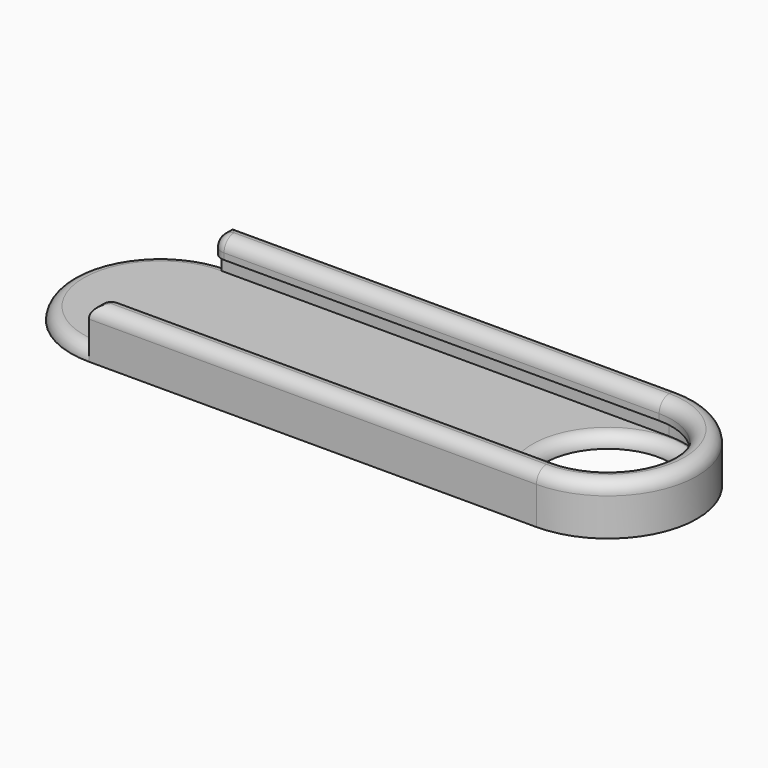
from build123d import *

# Parameters (mm, degrees)
F0_R         = 5
F1_DEPTH     = 1
F2_DEPTH     = 2.5
F4_DEPTH     = 1.5
F5_T1_DEPTH  = 35.75
F5_T3_DEPTH  = 1
F5_T5_DEPTH  = 34.75
F5_T7_DEPTH  = 1
F5_T9_DEPTH  = 0.5
F5_S13_W     = 1.02
F5_S13_H     = 1.02
F5_T14_DEPTH = 1.02
F5_S19_W     = 1.02
F5_S19_H     = 1.02
F5_T20_DEPTH = 1.02
F5_T24_ANGLE = 180
F5_T26_ANGLE = 180
F5_T30_ANGLE = 180
F5_T35_DEPTH = 3.5
F5_T39_DEPTH = 38.25
F5_T46_DEPTH = 38.25
F5_T50_DEPTH = 3.5


# Not quite as in the source:
# - a fillet or chamfer that OpenCascade refuses, or shapes differently, is made with other operations: its cross-section is extruded or revolved along the edge and cut away or added


with BuildPart() as f1:
    # F0 (on Top) → F1 (new body)
    with BuildSketch(Plane.XY):
        with BuildLine():
            Line((-12.4595724046, -6.125), (23.2904275954, -6.125))
            ThreePointArc((23.2904275954, -6.125), (29.4154275954, 0), (23.2904275954, 6.125))
            Line((23.2904275954, 6.125), (-12.4595724046, 6.125))
            ThreePointArc((-12.4595724046, 6.125), (-18.5845724046, 0), (-12.4595724046, -6.125))
        make_face()
        with Locations((23.2904275954, 0)):
            Circle(F0_R, mode=Mode.SUBTRACT)
        with BuildLine():
            Line((-12.4595724046, -7.125), (-12.4595724046, -6.125))
            ThreePointArc((-12.4595724046, -6.125), (-18.5845724046, 0), (-12.4595724046, 6.125))
            Line((-12.4595724046, 6.125), (-12.4595724046, 7.125))
            ThreePointArc((-12.4595724046, 7.125), (-19.5845724046, 0), (-12.4595724046, -7.125))
        make_face()
    extrude(amount=F1_DEPTH)

    # F0 (on Top) → F2 (join)
    with BuildSketch(Plane.XY):
        with BuildLine():
            ThreePointArc((23.2904275954, 6.125), (29.4154275954, 0), (23.2904275954, -6.125))
            Line((23.2904275954, -6.125), (-12.4595724046, -6.125))
            Line((-12.4595724046, -6.125), (-12.4595724046, -7.125))
            Line((-12.4595724046, -7.125), (23.2904275954, -7.125))
            ThreePointArc((23.2904275954, -7.125), (30.4154275954, 0), (23.2904275954, 7.125))
            Line((23.2904275954, 7.125), (-12.4595724046, 7.125))
            Line((-12.4595724046, 7.125), (-12.4595724046, 6.125))
            Line((-12.4595724046, 6.125), (23.2904275954, 6.125))
        make_face()
    extrude(amount=F2_DEPTH)

    # F3 (on face) → F4 (join)
    with BuildSketch(Plane.XY.offset(2.5)):
        with BuildLine():
            Line((-12.4595724046, -7.125), (23.2904275954, -7.125))
            ThreePointArc((23.2904275954, -7.125), (30.4154275954, 0), (23.2904275954, 7.125))
            Line((23.2904275954, 7.125), (-12.4595724046, 7.125))
            Line((-12.4595724046, 7.125), (-12.4595724046, 6.125))
            Line((-12.4595724046, 6.125), (23.2904275954, 6.125))
            ThreePointArc((23.2904275954, 6.125), (29.4154275954, 0), (23.2904275954, -6.125))
            Line((23.2904275954, -6.125), (-12.4595724046, -6.125))
            Line((-12.4595724046, -6.125), (-12.4595724046, -7.125))
        make_face()
        with BuildLine():
            Line((-12.4595724046, -5.125), (-12.4595724046, -6.125))
            Line((-12.4595724046, -6.125), (23.2904275954, -6.125))
            ThreePointArc((23.2904275954, -6.125), (29.4154275954, 0), (23.2904275954, 6.125))
            Line((23.2904275954, 6.125), (-12.4595724046, 6.125))
            Line((-12.4595724046, 6.125), (-12.4595724046, 5.125))
            Line((-12.4595724046, 5.125), (23.2904275954, 5.125))
            ThreePointArc((23.2904275954, 5.125), (28.4154275954, 0), (23.2904275954, -5.125))
            Line((23.2904275954, -5.125), (-12.4595724046, -5.125))
        make_face()
    extrude(amount=F4_DEPTH)

    # F5: fillet of radius 1 on 12 edges, made by hand

    # F5_s2 → F5_t1 (cut)
    with BuildSketch(Plane.YZ.offset(-12.4595724046)):
        with BuildLine():
            ThreePointArc((-6.125, 4), (-6.8321067812, 3.7071067812), (-7.125, 3))
            Line((-7.125, 3), (-7.145, 3))
            Line((-7.145, 3), (-7.145, 4.02))
            Line((-7.145, 4.02), (-6.125, 4.02))
            Line((-6.125, 4.02), (-6.125, 4))
        make_face()
        with BuildLine():
            ThreePointArc((6.125, 4), (6.8321067812, 3.7071067812), (7.125, 3))
            Line((7.125, 3), (7.145, 3))
            Line((7.145, 3), (7.145, 4.02))
            Line((7.145, 4.02), (6.125, 4.02))
            Line((6.125, 4.02), (6.125, 4))
        make_face()
    extrude(amount=F5_T1_DEPTH, mode=Mode.SUBTRACT)

    # F5_s4 → F5_t3 (cut)
    with BuildSketch(Plane.XZ.offset(-7.125)):
        with BuildLine():
            ThreePointArc((-11.4595724046, 4), (-12.1666791858, 3.7071067812), (-12.4595724046, 3))
            Line((-12.4595724046, 3), (-12.4795724046, 3))
            Line((-12.4795724046, 3), (-12.4795724046, 4.02))
            Line((-12.4795724046, 4.02), (-11.4595724046, 4.02))
            Line((-11.4595724046, 4.02), (-11.4595724046, 4))
        make_face()
    extrude(amount=F5_T3_DEPTH, mode=Mode.SUBTRACT)

    # F5_s6 → F5_t5 (cut)
    with BuildSketch(Plane.YZ.offset(-11.4595724046)):
        with BuildLine():
            ThreePointArc((6.125, 4), (5.4178932188, 3.7071067812), (5.125, 3))
            Line((5.125, 3), (5.105, 3))
            Line((5.105, 3), (5.105, 4.02))
            Line((5.105, 4.02), (6.125, 4.02))
            Line((6.125, 4.02), (6.125, 4))
        make_face()
        with BuildLine():
            ThreePointArc((-6.125, 4), (-5.4178932188, 3.7071067812), (-5.125, 3))
            Line((-5.125, 3), (-5.105, 3))
            Line((-5.105, 3), (-5.105, 4.02))
            Line((-5.105, 4.02), (-6.125, 4.02))
            Line((-6.125, 4.02), (-6.125, 4))
        make_face()
    extrude(amount=F5_T5_DEPTH, mode=Mode.SUBTRACT)

    # F5_s8 → F5_t7 (cut)
    with BuildSketch(Plane.XZ.offset(6.125)):
        with BuildLine():
            ThreePointArc((-12.4595724046, 3), (-12.1666791858, 3.7071067812), (-11.4595724046, 4))
            Line((-11.4595724046, 4), (-11.4595724046, 4.02))
            Line((-11.4595724046, 4.02), (-12.4795724046, 4.02))
            Line((-12.4795724046, 4.02), (-12.4795724046, 3))
            Line((-12.4795724046, 3), (-12.4595724046, 3))
        make_face()
    extrude(amount=F5_T7_DEPTH, mode=Mode.SUBTRACT)

    # F5_s10 → F5_t9 (cut)
    with BuildSketch(Plane.XY.offset(2.5)):
        with BuildLine():
            ThreePointArc((-12.4595724046, -6.125), (-12.1666791858, -5.4178932188), (-11.4595724046, -5.125))
            Line((-11.4595724046, -5.125), (-11.4595724046, -5.105))
            Line((-11.4595724046, -5.105), (-12.4795724046, -5.105))
            Line((-12.4795724046, -5.105), (-12.4795724046, -6.125))
            Line((-12.4795724046, -6.125), (-12.4595724046, -6.125))
        make_face()
        with BuildLine():
            ThreePointArc((-11.4595724046, 5.125), (-12.1666791858, 5.4178932188), (-12.4595724046, 6.125))
            Line((-12.4595724046, 6.125), (-12.4795724046, 6.125))
            Line((-12.4795724046, 6.125), (-12.4795724046, 5.105))
            Line((-12.4795724046, 5.105), (-11.4595724046, 5.105))
            Line((-11.4595724046, 5.105), (-11.4595724046, 5.125))
        make_face()
    extrude(amount=F5_T9_DEPTH, mode=Mode.SUBTRACT)


with BuildPart() as f5_tool12:
    # F5_s13 → F5_t14 (new body)
    with BuildSketch(Plane.YZ.offset(-11.4595724046)):
        with Locations((5.615, 3.51)):
            Rectangle(F5_S13_W, F5_S13_H)
    extrude(amount=-F5_T14_DEPTH)

    # F5_s15 → F5_t16 (revolve, cut)
    with BuildSketch(Plane(origin=(-11.4595724046, 6.125, 3), x_dir=(0, 0.7071067812, -0.7071067812), z_dir=(0, 0.7071067812, 0.7071067812))):
        with BuildLine():
            ThreePointArc((0, -1), (1, 0), (0, 1))
            Line((0, 1), (0, -1))
        make_face()
    revolve(axis=Axis((-11.4595724046, 6.125, 3), (-1, 0, 0)), mode=Mode.SUBTRACT)


with BuildPart() as f1_1:
    add(f1.part)

    # F5_t11: cut F5_tool12
    add(f5_tool12.part, mode=Mode.SUBTRACT)


with BuildPart() as f5_tool18:
    # F5_s19 → F5_t20 (new body)
    with BuildSketch(Plane.XZ.offset(6.125)):
        with Locations((-11.9695724046, 3.51)):
            Rectangle(F5_S19_W, F5_S19_H)
    extrude(amount=-F5_T20_DEPTH)

    # F5_s21 → F5_t22 (revolve, cut)
    with BuildSketch(Plane(origin=(-11.4595724046, -6.125, 3), x_dir=(0.7071067812, 0, -0.7071067812), z_dir=(0.7071067812, 0, 0.7071067812))):
        with BuildLine():
            ThreePointArc((0, -1), (1, 0), (0, 1))
            Line((0, 1), (0, -1))
        make_face()
    revolve(axis=Axis((-11.4595724046, -6.125, 3), (0, 1, 0)), mode=Mode.SUBTRACT)


with BuildPart() as f1_2:
    add(f1_1.part)

    # F5_t17: cut F5_tool18
    add(f5_tool18.part, mode=Mode.SUBTRACT)

    # F5_s23 → F5_t24 (revolve, cut)
    with BuildSketch(Plane.YZ.offset(23.2904275954)):
        with BuildLine():
            ThreePointArc((-6.125, 4), (-6.8321067812, 3.7071067812), (-7.125, 3))
            Line((-7.125, 3), (-7.145, 3))
            Line((-7.145, 3), (-7.145, 4.02))
            Line((-7.145, 4.02), (-6.125, 4.02))
            Line((-6.125, 4.02), (-6.125, 4))
        make_face()
    revolve(axis=Axis((23.2904275954, 0, 4), (0, 0, 1)), revolution_arc=F5_T24_ANGLE, mode=Mode.SUBTRACT)

    # F5_s25 → F5_t26 (revolve, cut)
    with BuildSketch(Plane.YZ.offset(23.2904275954)):
        with BuildLine():
            ThreePointArc((6.125, 4), (5.4178932188, 3.7071067812), (5.125, 3))
            Line((5.125, 3), (5.105, 3))
            Line((5.105, 3), (5.105, 4.02))
            Line((5.105, 4.02), (6.125, 4.02))
            Line((6.125, 4.02), (6.125, 4))
        make_face()
    revolve(axis=Axis((23.2904275954, 0, 4), (0, 0, -1)), revolution_arc=F5_T26_ANGLE, mode=Mode.SUBTRACT)

    # F5_s27 → F5_t28 (revolve, cut)
    with BuildSketch(Plane.XZ):
        with BuildLine():
            ThreePointArc((29.2904275954, 1), (28.5833208142, 0.7071067812), (28.2904275954, 0))
            Line((28.2904275954, 0), (28.2704275954, 0))
            Line((28.2704275954, 0), (28.2704275954, 1.02))
            Line((28.2704275954, 1.02), (29.2904275954, 1.02))
            Line((29.2904275954, 1.02), (29.2904275954, 1))
        make_face()
    revolve(axis=Axis((23.2904275954, 0, 1), (0, 0, 1)), mode=Mode.SUBTRACT)

    # F5_s29 → F5_t30 (revolve, cut)
    with BuildSketch(Plane.YZ.offset(-12.4595724046)):
        with BuildLine():
            ThreePointArc((7.125, 0), (6.8321067812, 0.7071067812), (6.125, 1))
            Line((6.125, 1), (6.125, 1.02))
            Line((6.125, 1.02), (7.145, 1.02))
            Line((7.145, 1.02), (7.145, 0))
            Line((7.145, 0), (7.125, 0))
        make_face()
    revolve(axis=Axis((-12.4595724046, 0, 1), (0, 0, 1)), revolution_arc=F5_T30_ANGLE, mode=Mode.SUBTRACT)


with BuildPart() as f5_tool33:
    # F5_s34 → F5_t35 (new body)
    with BuildSketch(Plane.XZ.offset(6.125)):
        with BuildLine():
            ThreePointArc((-12.4595724046, 3), (-12.1666791858, 3.7071067812), (-11.4595724046, 4))
            Line((-11.4595724046, 4), (-11.4595724046, 4.02))
            Line((-11.4595724046, 4.02), (-12.4795724046, 4.02))
            Line((-12.4795724046, 4.02), (-12.4795724046, 3))
            Line((-12.4795724046, 3), (-12.4595724046, 3))
        make_face()
    extrude(amount=F5_T35_DEPTH)

    split(bisect_by=Plane.XZ.offset(7.125), keep=Keep.TOP)


with BuildPart() as f5_tool37:
    # F5_s38 → F5_t39 (new body)
    with BuildSketch(Plane.YZ.offset(-14.9595724046)):
        with BuildLine():
            ThreePointArc((-6.125, 4), (-6.8321067812, 3.7071067812), (-7.125, 3))
            Line((-7.125, 3), (-7.145, 3))
            Line((-7.145, 3), (-7.145, 4.02))
            Line((-7.145, 4.02), (-6.125, 4.02))
            Line((-6.125, 4.02), (-6.125, 4))
        make_face()
    extrude(amount=F5_T39_DEPTH)

    split(bisect_by=Plane.YZ.offset(-12.4595724046), keep=Keep.BOTTOM)


with BuildPart() as f5_tool33_1:
    add(f5_tool33.part)

    # F5_t41: intersect F5_tool37
    add(f5_tool37.part, mode=Mode.INTERSECT)


with BuildPart() as f1_3:
    add(f1_2.part)

    # F5_t31: cut F5_tool33
    add(f5_tool33_1.part, mode=Mode.SUBTRACT)


with BuildPart() as f5_tool44:
    # F5_s45 → F5_t46 (new body)
    with BuildSketch(Plane.YZ.offset(23.2904275954)):
        with BuildLine():
            ThreePointArc((6.125, 4), (6.8321067812, 3.7071067812), (7.125, 3))
            Line((7.125, 3), (7.145, 3))
            Line((7.145, 3), (7.145, 4.02))
            Line((7.145, 4.02), (6.125, 4.02))
            Line((6.125, 4.02), (6.125, 4))
        make_face()
    extrude(amount=-F5_T46_DEPTH)

    split(bisect_by=Plane.YZ.offset(-12.4595724046), keep=Keep.BOTTOM)


with BuildPart() as f5_tool48:
    # F5_s49 → F5_t50 (new body)
    with BuildSketch(Plane.XZ.offset(-9.625)):
        with BuildLine():
            ThreePointArc((-11.4595724046, 4), (-12.1666791858, 3.7071067812), (-12.4595724046, 3))
            Line((-12.4595724046, 3), (-12.4795724046, 3))
            Line((-12.4795724046, 3), (-12.4795724046, 4.02))
            Line((-12.4795724046, 4.02), (-11.4595724046, 4.02))
            Line((-11.4595724046, 4.02), (-11.4595724046, 4))
        make_face()
    extrude(amount=F5_T50_DEPTH)

    split(bisect_by=Plane.XZ.offset(-7.125), keep=Keep.BOTTOM)


with BuildPart() as f5_tool44_1:
    add(f5_tool44.part)

    # F5_t52: intersect F5_tool48
    add(f5_tool48.part, mode=Mode.INTERSECT)


with BuildPart() as f1_4:
    add(f1_3.part)

    # F5_t42: cut F5_tool44
    add(f5_tool44_1.part, mode=Mode.SUBTRACT)


solid = f1_4.part
